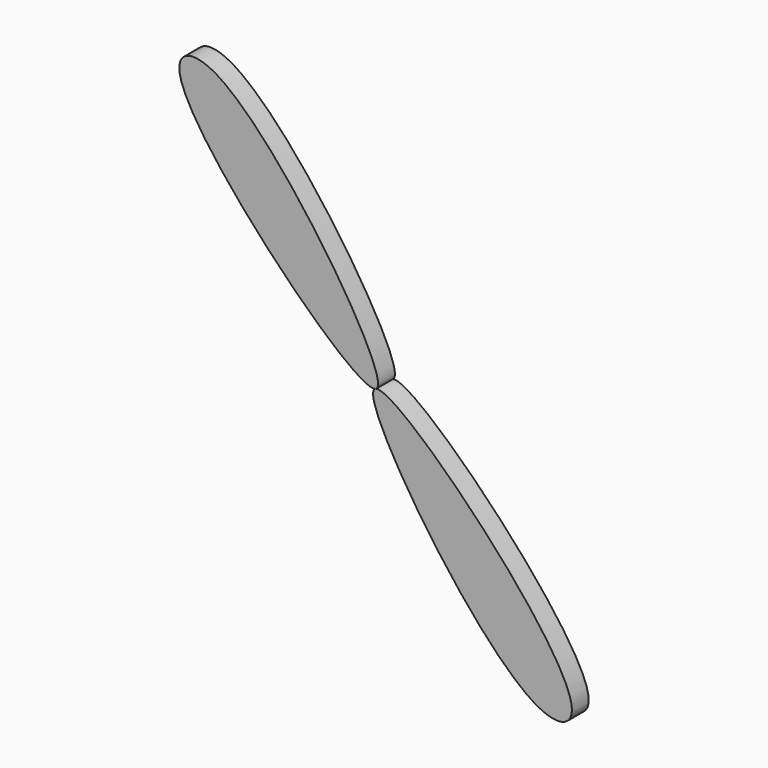
from build123d import *

# Parameters (mm, degrees)
F1_DEPTH = 12.7


# Not quite as in the source:
# - ends of sketch curves that miss each other by under 0.0002 mm in the source are joined


with BuildPart() as f1:
    # F0 (on Front) → F1 (new body)
    with BuildSketch(Plane.XZ):
        with BuildLine():
            add(Edge.make_bspline(
                [(0.0851461084, 0.0364977736), (13.4173432124, 4.981764724), (147.1814805715, -130.9795197626), (84.5685821352, -154.1438118144), (-12.3258406715, -6.0428114175), (-0.1248385092, -0.0535120943)],
                knots=[0.0023124215, 0.0023124215, 0.0023124215, 0.0023124215, 0.4274724605, 0.581813776, 1, 1, 1, 1], degree=3))
            add(Edge.make_bspline(
                [(0.0851461084, 0.0364977736), (0.0176790191, 0.003378732), (-0.0523253132, -0.0266154056), (-0.1248385092, -0.0535120943)],
                knots=[0, 0, 0, 0, 0.0023124215, 0.0023124215, 0.0023124215, 0.0023124215], degree=3))
        make_face()
        with BuildLine():
            add(Edge.make_bspline(
                [(-0.1248385092, -0.0535120943), (-0.0573712937, -0.0203933929), (0.0126330385, 0.0096007449), (0.0851461084, 0.0364977736)],
                knots=[0, 0, 0, 0, 0.0023124215, 0.0023124215, 0.0023124215, 0.0023124215], degree=3))
            add(Edge.make_bspline(
                [(-0.1248385092, -0.0535120943), (-13.4570356208, -4.9987794155), (-147.2211737889, 130.9625055247), (-84.608274516, 154.1267975242), (12.2861485254, 6.0257967738), (0.0851461084, 0.0364977736)],
                knots=[0.0023124215, 0.0023124215, 0.0023124215, 0.0023124215, 0.4274724602, 0.5818137766, 1, 1, 1, 1], degree=3))
        make_face()
        with BuildLine():
            add(Edge.make_bspline(
                [(0.0851462346, 0.0364974332), (0.0176790191, 0.003378732), (-0.0523253132, -0.0266154056), (-0.1248383831, -0.0535124342)],
                knots=[0, 0, 0, 0, 0.0023124215, 0.0023124215, 0.0023124215, 0.0023124215], degree=3))
            add(Edge.make_bspline(
                [(-0.1248383831, -0.0535124342), (-0.0573712937, -0.0203933929), (0.0126330385, 0.0096007449), (0.0851462346, 0.0364974332)],
                knots=[0, 0, 0, 0, 0.0023124215, 0.0023124215, 0.0023124215, 0.0023124215], degree=3))
        make_face()
    extrude(amount=F1_DEPTH)


solid = f1.part
